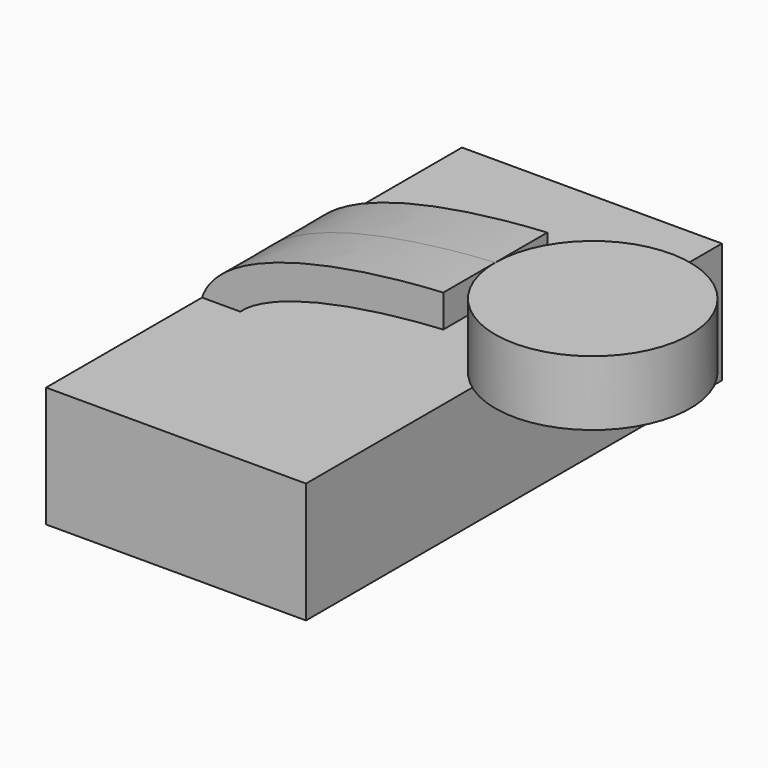
from build123d import *

# Parameters (mm, degrees)
F1_DEPTH = 76.2
F3_DEPTH = 19.05


# Not quite as in the source:
# - the dataset's text gives a spline's control points without its knots; the knots are read off the source's solid


with BuildPart() as f1:
    # F0 (on Front) → F1 (new body, symmetric)
    with BuildSketch(Plane.XZ):
        Polygon((-38.1, -17.6673417512), (38.1, -17.6673417512), (38.1, 17.6673417512), (-26.8917303536, 17.6673417512), (-38.1, 17.6673417512), align=None)
    extrude(amount=F1_DEPTH, both=True)

    # F0 (on Front) → F3 (join, symmetric)
    with BuildSketch(Plane.XZ):
        with BuildLine():
            add(Edge.make_bspline(
                [(-38.1, 17.6673417512), (-31.8581272554, 36.410088553), (15.1040040718, 41.0189594396), (32.6177167096, 41.9407316055)],
                knots=[0, 0, 0, 0, 74.7675926565, 74.7675926565, 74.7675926565, 74.7675926565], degree=3))
            Line((-38.1, 17.6673417512), (-26.8917303536, 17.6673417512))
            add(Edge.make_bspline(
                [(-26.8917303536, 17.6673417512), (-26.407134676, 18.1192768496), (-25.1094875132, 19.1894372172), (-22.3798521949, 20.9176688703), (-18.7227956487, 22.7186175127), (-13.0549393733, 24.9573096618), (-4.8316945698, 27.3548737), (5.8399746203, 29.5213200126), (16.3861493136, 31.034333018), (25.6713292387, 31.9611156892), (30.6234236258, 32.2921996469), (32.6177167096, 32.4019445138)],
                knots=[0.1376234231, 0.1376234231, 0.1376234231, 0.1376234231, 0.1875, 0.25, 0.3125, 0.375, 0.5, 0.625, 0.75, 0.875, 0.9902000327, 0.9902000327, 0.9902000327, 0.9902000327], degree=3))
            Line((32.6177167096, 32.4019445138), (32.6177167096, 41.9407316055))
        make_face()
    extrude(amount=F3_DEPTH, both=True)


with BuildPart() as f2:
    # F0 (on Front) → F2 (revolve)
    with BuildSketch(Plane.XZ):
        Polygon((61.1927167096, 41.9407316055), (32.6177167096, 41.9407316055), (32.6177167096, 32.4019445138), (32.6177167096, 22.8907316055), (61.1927167096, 22.8907316055), align=None)
    revolve(axis=Axis((61.1927167096, 0, 32.4157316055), (0, 0, 1)))


solid = Compound([f1.part, f2.part])
